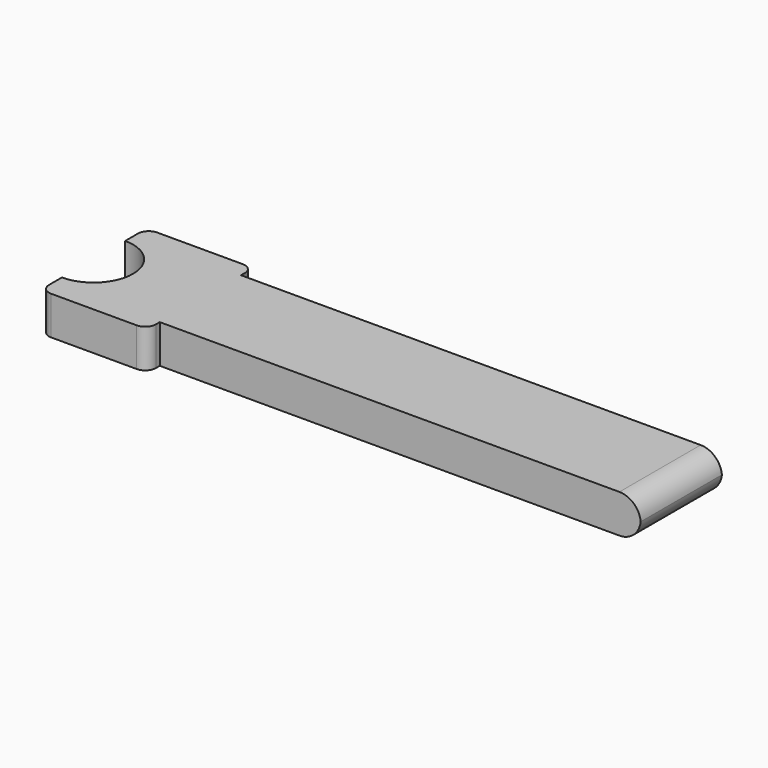
from build123d import *

# Parameters (mm, degrees)
F1_DEPTH    = 9.144
F2_R        = 2.54
F3_W        = 24.13
F3_H        = 9.144
F4_DEPTH    = 114.3
F5_T1_DEPTH = 49.53


# Not quite as in the source:
# - a fillet or chamfer that OpenCascade refuses, or shapes differently, is made with other operations: its cross-section is extruded or revolved along the edge and cut away or added


with BuildPart() as f1:
    # F0 (on Top) → F1 (new body)
    with BuildSketch(Plane.XY):
        with BuildLine():
            ThreePointArc((0, 9.398), (9.398, 0), (0, -9.398))
            Line((0, -9.398), (0, -15.748))
            Line((0, -15.748), (25.4, -15.748))
            Line((25.4, -15.748), (25.4, 15.748))
            Line((25.4, 15.748), (0, 15.748))
            Line((0, 15.748), (0, 9.398))
        make_face()
    extrude(amount=F1_DEPTH)

    # F2
    f2_edges = [f1.edges().sort_by_distance(p)[0] for p in [
        (25.4, -15.748, 4.572),
        (0, -15.748, 4.572),
        (0, 15.748, 4.572),
        (25.4, 15.748, 4.572),
    ]]
    fillet(f2_edges, radius=F2_R)

    # F3 (on face) → F4 (join)
    with BuildSketch(Plane.YZ.offset(25.4)):
        with Locations((0, 4.572)):
            Rectangle(F3_W, F3_H)
    extrude(amount=F4_DEPTH)

    # F5: fillet of radius 5.08 on 2 edges, made by hand

    # F5_s2 → F5_t1 (cut)
    with BuildSketch(Plane.XZ.offset(-24.765)):
        with BuildLine():
            ThreePointArc((134.62, 9.144), (138.2121024484, 7.6561024484), (139.7, 4.064))
            Line((139.7, 4.064), (139.7, 9.144))
            Line((139.7, 9.144), (134.62, 9.144))
        make_face()
        with BuildLine():
            ThreePointArc((134.62, 0), (138.2121024484, 1.4878975516), (139.7, 5.08))
            Line((139.7, 5.08), (139.7, 0))
            Line((139.7, 0), (134.62, 0))
        make_face()
    extrude(amount=F5_T1_DEPTH, mode=Mode.SUBTRACT)


solid = f1.part
